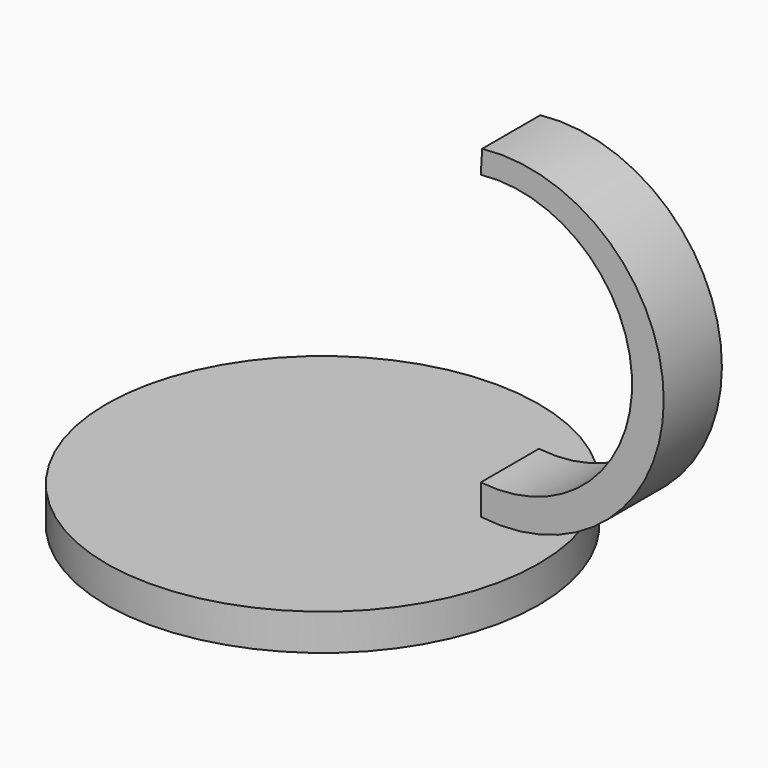
from build123d import *

# Parameters (mm, degrees)
F3_DEPTH = 10
F4_R     = 29.7263240479
F5_DEPTH = 5


# Not quite as in the source:
# - the program builds the solid bodies; features that only make, move or delete a surface that nothing else refers to are left out


with BuildPart() as f3:
    # F2 (on Front) → F3 (new body)
    with BuildSketch(Plane.XZ):
        with BuildLine():
            Line((29.749751091, 18.9209990203), (29.749751091, 14.7464834154))
            ThreePointArc((29.749751091, 14.7464834154), (54.9120135043, 36.9502850693), (29.9429353327, 59.3711100519))
            Line((29.9429353327, 59.3711100519), (29.749751091, 56.1637170613))
            ThreePointArc((29.749751091, 56.1637170613), (50.5571184209, 37.5423580408), (29.749751091, 18.9209990203))
        make_face()
    extrude(amount=F3_DEPTH)


with BuildPart() as f5:
    # F4 (on Top) → F5 (new body)
    with BuildSketch(Plane.XY):
        Circle(F4_R)
    extrude(amount=F5_DEPTH)


solid = Compound([f3.part, f5.part])
